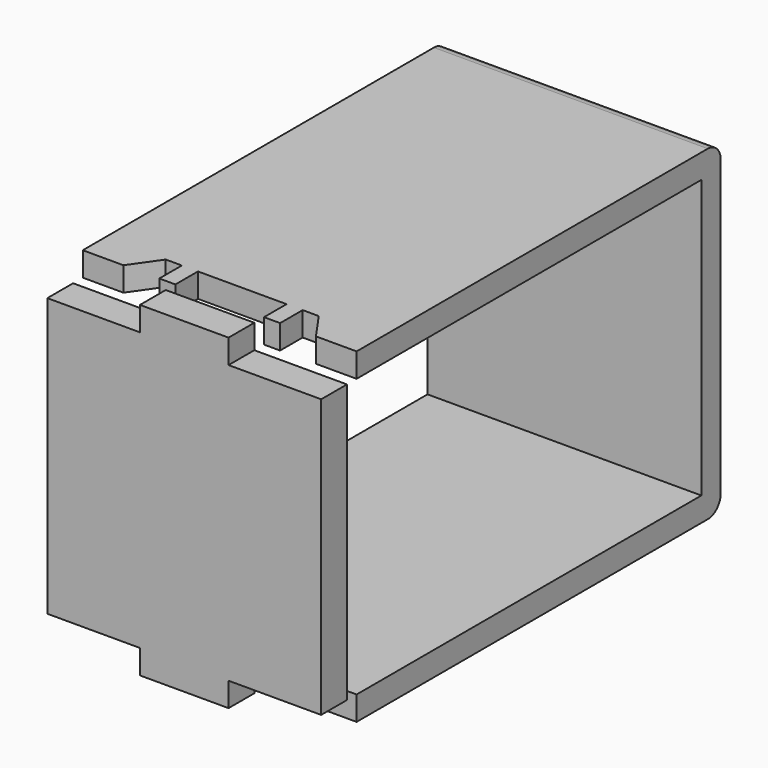
from build123d import *

# Parameters (mm, degrees)
F5_DEPTH  = 3
F7_W      = 34
F7_H      = 40.5
F8_DEPTH  = 3
F9_R      = 2
F11_W     = 11
F11_H     = 3
F12_DEPTH = 4


with BuildPart() as f5:
    # F2 (on Top) → F5 (new body)
    with BuildSketch(Plane.XY):
        Polygon((-17, 26.75), (-17, -26.75), (-11.9507263837, -26.75), (-9.5, -23.25), (-7.5, -23.25), (-7.5, -26.75), (-5.5, -26.75), (-5.5, -23.25), (5.5, -23.25), (5.5, -26.75), (7.5, -26.75), (7.5, -23.25), (9.5, -23.25), (11.9507263837, -26.75), (17, -26.75), (17, 26.75), align=None)
    extrude(amount=F5_DEPTH)



with BuildPart() as f5b:
    # F4 (on offset) → F5, piece 2 (new body)
    with BuildSketch(Plane.XY.offset(37.5)):
        Polygon((5.5, -26.75), (7.5, -26.75), (7.5, -23.25), (9.5, -23.25), (11.9507263837, -26.75), (17, -26.75), (17, 26.75), (-17, 26.75), (-17, -26.75), (-11.9507263837, -26.75), (-9.5, -23.25), (-7.5, -23.25), (-7.5, -26.75), (-5.5, -26.75), (-5.5, -23.25), (5.5, -23.25), align=None)
    extrude(amount=F5_DEPTH)


with BuildPart() as f5_1:
    add(f5.part)

    add(f5b.part)  # F8 merges F5b
    # F7 (on offset) → F8 (join)
    with BuildSketch(Plane(origin=(0, 26.75, 0), x_dir=(-1, 0, 0), z_dir=(0, 1, 0))):
        with Locations((0, 20.25)):
            Rectangle(F7_W, F7_H)
    extrude(amount=F8_DEPTH)

    # F9
    f9_edges = [f5_1.edges().sort_by_distance(p)[0] for p in [
        (0, 29.75, 40.5),
        (0, 29.75, 0),
    ]]
    fillet(f9_edges, radius=F9_R)


with BuildPart() as f12:
    # F11 (on offset) → F12 (new body)
    with BuildSketch(Plane.XZ.offset(28.25)):
        with Locations((0, 39)):
            Rectangle(F11_W, F11_H)
        Polygon((5.5, 37.5), (-5.5, 37.5), (-17, 37.5), (-17, 3), (-5.5, 3), (5.5, 3), (17, 3), (17, 37.5), align=None)
        with Locations((0, 1.5)):
            Rectangle(F11_W, F11_H)
    extrude(amount=F12_DEPTH)


solid = Compound([f5_1.part, f12.part])
